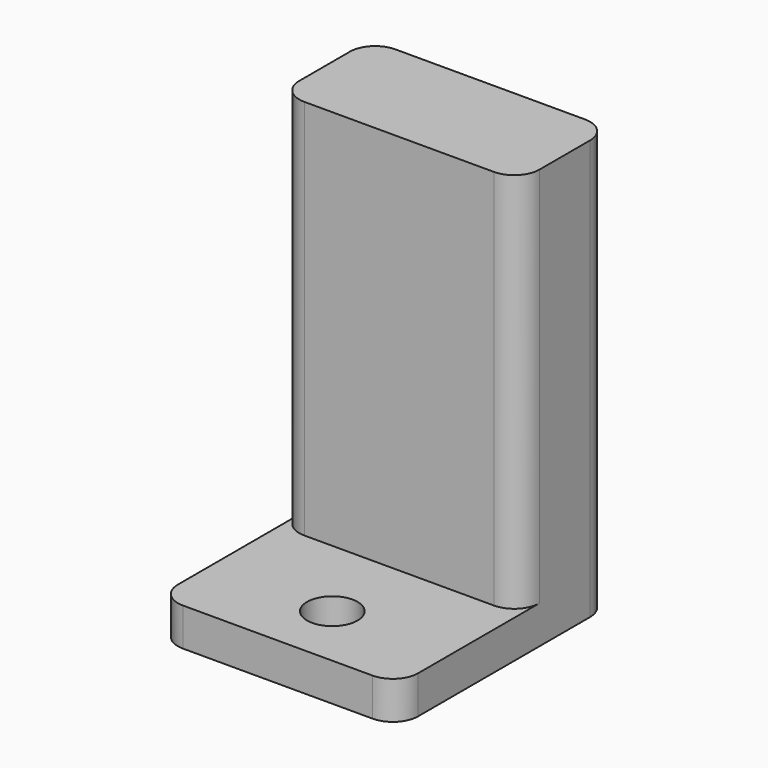
from build123d import *

# Parameters (mm, degrees)
F0_W     = 16
F0_H     = 8
F1_DEPTH = 8
F2_W     = 16
F2_H     = 3
F3_DEPTH = 33.2
F4_W     = 19
F4_H     = 3
F5_DEPTH = 12
F6_R     = 2
F7_DEPTH = 3
F8_W     = 16
F8_H     = 3
F9_DEPTH = 6
F10_R    = 1.99999


# Not quite as in the source:
# - a fillet or chamfer is up to 0.001 mm smaller than in the source, because OpenCascade refuses the exact size


with BuildPart() as f1:
    # F0 (on Top) → F1 (new body)
    with BuildSketch(Plane.XY):
        with Locations((-8, 4)):
            Rectangle(F0_W, F0_H)
    extrude(amount=F1_DEPTH)

    # F2 (on Top) → F3 (join)
    with BuildSketch(Plane.XY):
        with Locations((-8, -1.5)):
            Rectangle(F2_W, F2_H)
        Polygon((0, 6), (0, 0), (0, -3), (3, -3), (3, 6), align=None)
    extrude(amount=F3_DEPTH)

    # F4 (on face) → F5 (join)
    with BuildSketch(Plane.XZ.offset(3)):
        with Locations((-6.5, 1.5)):
            Rectangle(F4_W, F4_H)
    extrude(amount=F5_DEPTH)

    # F6 (on face) → F7 (cut, through all)
    with BuildSketch(Plane.XY.offset(3)):
        with Locations((-6.3249543309, -9.8292976618)):
            Circle(F6_R)
    extrude(amount=-F7_DEPTH, mode=Mode.SUBTRACT)

    # F8 (on face) → F9 (join)
    with BuildSketch(Plane(origin=(0, 0, 0), x_dir=(-1, 0, 0), z_dir=(0, 1, 0))):
        with Locations((8, 31.7)):
            Rectangle(F8_W, F8_H)
    extrude(amount=F9_DEPTH)

    # F10 (radius 2 in the source; OpenCascade refuses exactly that, so slightly less here)
    f10_edges = [f1.edges().sort_by_distance(p)[0] for p in [
        (-16, 6, 31.7),
        (-16, 8, 4),
        (0, 8, 4),
        (3, 6, 16.6),
        (3, -15, 1.5),
        (3, -3, 18.1),
        (-16, -3, 18.1),
        (-16, -15, 1.5),
    ]]
    fillet(f10_edges, radius=F10_R)


solid = f1.part
